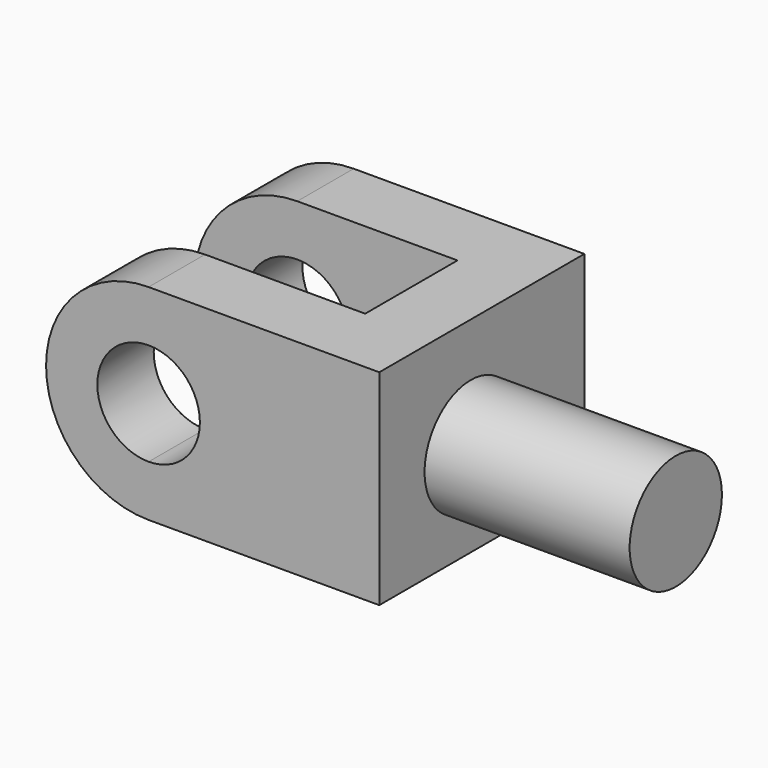
from build123d import *
from build123d import SkipClean  # not in build123d's __all__

# Parameters (mm, degrees)
F0_R      = 228.6
F1_DEPTH  = 812.8
F0_W      = 1016
F0_H      = 812.8
F1_FACE_R = 228.6
F2_DEPTH  = 914.4
F4_DEPTH  = 279.4
F6_DEPTH  = 1016.001
F7_W      = 635
F7_H      = 457.2
F8_DEPTH  = 812.801
F10_DEPTH = 279.4


# Not quite as in the source:
# - after a boolean that leaves OpenCascade's solid faulty, fix() repairs it


with BuildPart() as f1:
    # F0 (on Right) → F1 (new body)
    with BuildSketch(Plane.YZ):
        with Locations((330.030798912, 303.7791848183)):
            Circle(F0_R)
    extrude(amount=F1_DEPTH)

    # F0 (on Right) + F1_face (on face) → F2 (join)
    with BuildSketch(Plane.YZ):
        with Locations((384.9944980741, 337.2235123754)):
            Rectangle(F0_W, F0_H)
        with Locations((330.030798912, 303.7791848183)):
            Circle(F0_R, mode=Mode.SUBTRACT)
    with BuildSketch(Plane(origin=(0, 330.030798912, 303.7791848183), x_dir=(0, 1, 0), z_dir=(-1, 0, 0))):
        Circle(F1_FACE_R)
    extrude(amount=-F2_DEPTH, dir=(1, 0, 0))

    # F3 (on face) → F4 (join)
    with BuildSketch(Plane.XZ.offset(123.0055019259)):
        with BuildLine():
            ThreePointArc((-914.4, 743.6235123754), (-1320.8, 337.2235123754), (-914.4, -69.1764876246))
            Line((-914.4, -69.1764876246), (-914.4, 134.0235123754))
            ThreePointArc((-914.4, 134.0235123754), (-1117.6, 337.2235123754), (-914.4, 540.4235123754))
            Line((-914.4, 540.4235123754), (-914.4, 743.6235123754))
        make_face()
    extrude(amount=-F4_DEPTH)

    # F5 (on face) → F6 (cut, through all)
    with BuildSketch(Plane.XZ.offset(123.0055019259)):
        with BuildLine():
            Line((-914.4, 540.4235123754), (-914.4, 134.0235123754))
            ThreePointArc((-914.4, 134.0235123754), (-770.7159020629, 193.5394144382), (-711.2, 337.2235123754))
            ThreePointArc((-711.2, 337.2235123754), (-770.7159020629, 480.9076103125), (-914.4, 540.4235123754))
        make_face()
    with SkipClean():  # cleaning this boolean's faces spoils the solid; the shape is the same uncleaned
        extrude(amount=-F6_DEPTH, mode=Mode.SUBTRACT)

    # F7 (on face) → F8 (cut, through all)
    with BuildSketch(Plane.XY.offset(743.6235123754)):
        with Locations((-596.9, 384.9944980741)):
            Rectangle(F7_W, F7_H)
    extrude(amount=-F8_DEPTH, mode=Mode.SUBTRACT)

    add(f1.part.fix(), mode=Mode.REPLACE)

    # F9 (on face) → F10 (join)
    with BuildSketch(Plane.XZ.offset(-613.5944980741)):
        with BuildLine():
            Line((-914.4, 540.4235123754), (-914.4, 743.6235123754))
            ThreePointArc((-914.4, 743.6235123754), (-1320.8, 337.2235123754), (-914.4, -69.1764876246))
            Line((-914.4, -69.1764876246), (-914.4, 134.0235123754))
            ThreePointArc((-914.4, 134.0235123754), (-1117.6, 337.2235123754), (-914.4, 540.4235123754))
        make_face()
    extrude(amount=-F10_DEPTH)


solid = f1.part
